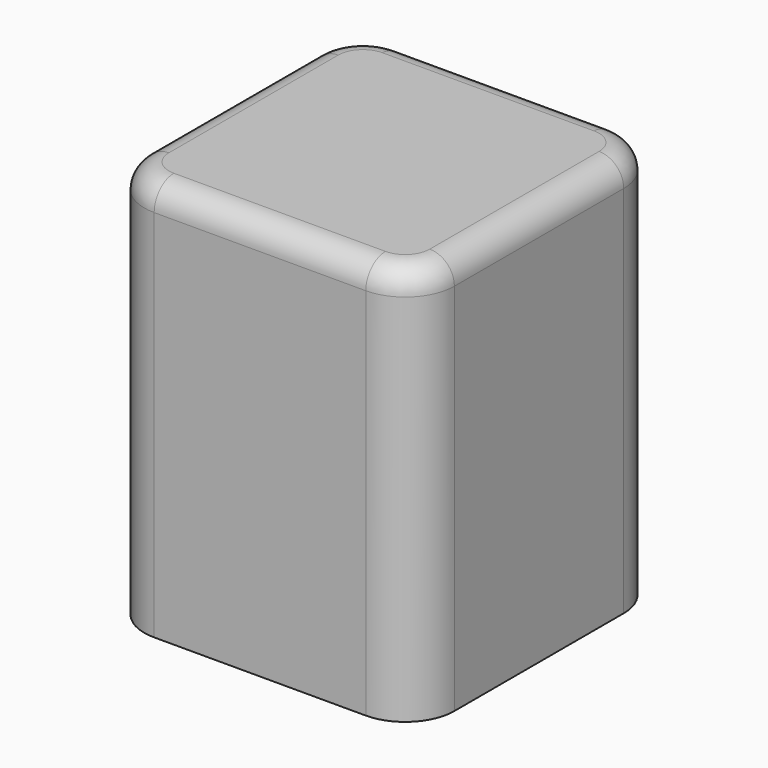
from build123d import *

# Parameters (mm, degrees)
F0_W         = 63
F0_H         = 63
F1_DEPTH     = 81
F2_W         = 53
F2_H         = 53
F3_DEPTH     = 76
F4_R         = 1
F5_DEPTH     = 10
F6_R         = 10
F7_R         = 5
F8_TEXT_SIZE = 19.0531513215
F9_DEPTH     = 1


# Not quite as in the source:
# - Text() gives the source's letters only with a copy of the font that has no kerning and outlines rounded to 1/6400 em; it was checked with that copy


with BuildPart() as f1:
    # F0 (on Top) → F1 (new body)
    with BuildSketch(Plane.XY):
        Rectangle(F0_W, F0_H)
    extrude(amount=F1_DEPTH)

    # F2 (on face) → F3 (cut, through all)
    with BuildSketch(Plane(origin=(0, 0, 0), x_dir=(1, 0, 0), z_dir=(0, 0, -1))):
        Rectangle(F2_W, F2_H)
    extrude(amount=-F3_DEPTH, mode=Mode.SUBTRACT)

    # F4 (on face) → F5 (cut)
    with BuildSketch(Plane(origin=(0, 0, 0), x_dir=(1, 0, 0), z_dir=(0, 0, -1))):
        with Locations((-29, 0)):
            Circle(F4_R)
        with Locations((0, 29)):
            Circle(F4_R)
        with Locations((29, 0)):
            Circle(F4_R)
        with Locations((0, -29)):
            Circle(F4_R)
    extrude(amount=-F5_DEPTH, mode=Mode.SUBTRACT)

    # F6
    f6_edges = [f1.edges().sort_by_distance(p)[0] for p in [
        (-31.5, -31.5, 40.5),
        (-31.5, 31.5, 40.5),
        (31.5, 31.5, 40.5),
        (31.5, -31.5, 40.5),
    ]]
    fillet(f6_edges, radius=F6_R)

    # F7
    f7_edges = [f1.edges().sort_by_distance(p)[0] for p in [
        (0, -31.5, 81),
        (-28.571068, -28.571068, 81),
        (28.571068, -28.571068, 81),
        (-31.5, 0, 81),
        (31.5, 0, 81),
        (-28.571068, 28.571068, 81),
        (28.571068, 28.571068, 81),
        (0, 31.5, 81),
    ]]
    fillet(f7_edges, radius=F7_R)

    # F8 (on face) → F9 (cut)
    with BuildSketch(Plane(origin=(0, 31.5, 0), x_dir=(-1, 0, 0), z_dir=(0, 1, 0))):
        with Locations((-20.5, 12)):
            Text('BOB', F8_TEXT_SIZE, font='Open Sans', font_style=FontStyle.BOLD, text_align=(TextAlign.LEFT, TextAlign.BOTTOM))
    extrude(amount=-F9_DEPTH, mode=Mode.SUBTRACT)


solid = f1.part
